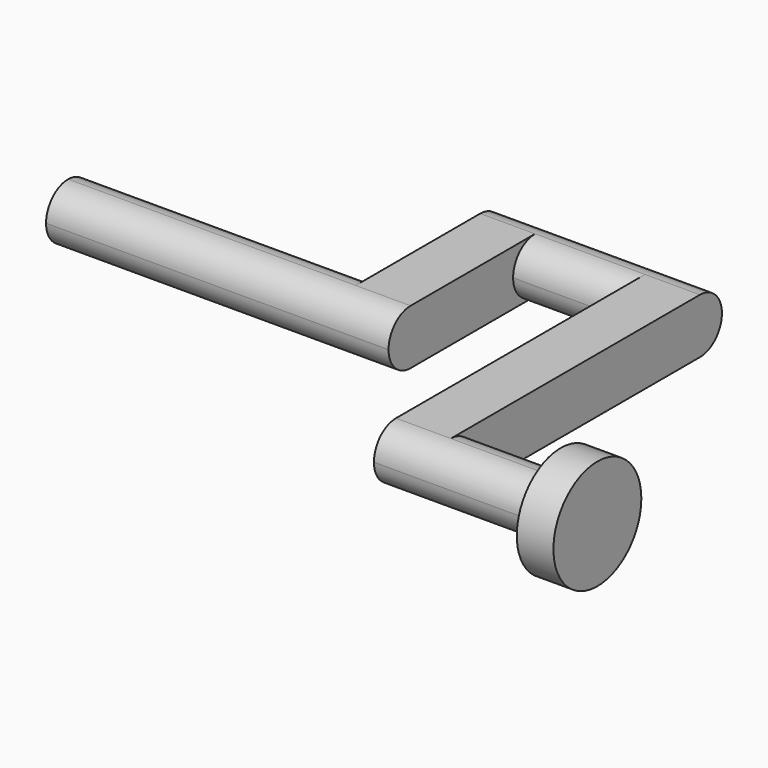
from build123d import *

# Parameters (mm, degrees)
F1_DEPTH = 3.81
F2_R     = 1.90499
F3_R     = 3.81
F4_DEPTH = 2.54


# Not quite as in the source:
# - a fillet or chamfer is up to 0.001 mm smaller than in the source, because OpenCascade refuses the exact size
# - ends of sketch curves that miss each other by under 0.0002 mm in the source are joined


with BuildPart() as f1:
    # F0 (on Top) → F1 (new body)
    with BuildSketch(Plane.XY):
        Polygon((19.939, 0), (0, 0), (0, -3.81), (23.749, -3.81), (23.749, 6.985), (31.369, 6.985), (31.369, -14.605), (42.799, -14.605), (42.799, -10.795), (35.179, -10.795), (35.179, 10.795), (19.939, 10.795), align=None)
    extrude(amount=F1_DEPTH)

    # F2 (radius 1.905 in the source; OpenCascade refuses exactly that, so slightly less here)
    f2_edges = [f1.edges().sort_by_distance(p)[0] for p in [
        (9.9695, 0, 3.81),
        (9.9695, 0, 0),
        (11.8745, -3.81, 3.81),
        (11.8745, -3.81, 0),
        (27.559, 10.795, 3.81),
        (27.559, 6.985, 3.81),
        (27.559, 6.985, 0),
        (27.559, 10.795, 0),
        (38.989, -10.795, 3.81),
        (37.084, -14.605, 3.81),
        (38.989, -10.795, 0),
        (37.084, -14.605, 0),
    ]]
    fillet(f2_edges, radius=F2_R)

    # F3 (on face) → F4 (join)
    with BuildSketch(Plane.YZ.offset(42.799)):
        with Locations((-12.7, 1.905)):
            Circle(F3_R)
        with BuildLine():
            ThreePointArc((-12.70001, 0), (-14.0470413471, 0.5579586529), (-14.605, 1.90499))
            ThreePointArc((-14.605, 1.90499), (-14.0470413471, 3.2520413471), (-12.70001, 3.81))
            ThreePointArc((-12.70001, 3.81), (-11.3529586529, 3.2520413471), (-10.795, 1.90501))
            ThreePointArc((-10.795, 1.90501), (-11.3529586529, 0.5579586529), (-12.70001, 0))
        make_face(mode=Mode.SUBTRACT)
        with BuildLine():
            ThreePointArc((-12.70001, 3.81), (-14.0470413471, 3.2520413471), (-14.605, 1.90501))
            ThreePointArc((-14.605, 1.90501), (-14.0470413471, 0.5579586529), (-12.70001, 0))
            ThreePointArc((-12.70001, 0), (-11.3529586529, 0.5579586529), (-10.795, 1.90499))
            ThreePointArc((-10.795, 1.90499), (-11.3529586529, 3.2520413471), (-12.70001, 3.81))
        make_face()
    extrude(amount=F4_DEPTH)


solid = f1.part
